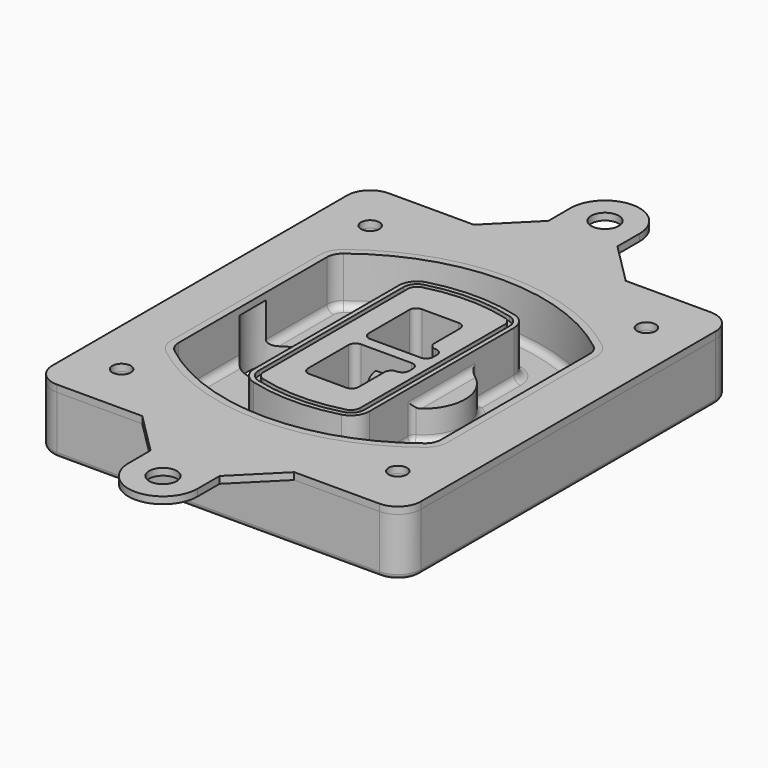
from build123d import *

# Parameters (mm, degrees)
F0_R      = 4
F1_DEPTH  = 25
F2_DEPTH  = 3
F3_DEPTH  = 18
F5_DEPTH  = 21
F6_DEPTH  = 2
F8_DEPTH  = 20
F9_DEPTH  = 16
F10_DEPTH = 25
F7_R      = 6
F7_R_2    = 4
F11_DEPTH = 6
F13_DEPTH = 9
F14_R     = 3
F15_R     = 2
F16_R     = 4
F16_R_2   = 6
F17_DEPTH = 3


# Not quite as in the source:
# - ends of sketch curves that miss each other by under 0.0002 mm in the source are joined


with BuildPart() as f1:
    # F0 (on Top) → F1 (new body)
    with BuildSketch(Plane.XY):
        with BuildLine():
            ThreePointArc((-80, -80), (-77.0710678119, -87.0710678119), (-70, -90))
            Line((-70, -90), (70, -90))
            ThreePointArc((70, -90), (77.0710678119, -87.0710678119), (80, -80))
            Line((80, -80), (80, 80))
            ThreePointArc((80, 80), (77.0710678119, 87.0710678119), (70, 90))
            Line((70, 90), (-70, 90))
            ThreePointArc((-70, 90), (-77.0710678119, 87.0710678119), (-80, 80))
            Line((-80, 80), (-80, -80))
        make_face()
        with Locations((-60, -67.5)):
            Circle(F0_R, mode=Mode.SUBTRACT)
        with Locations((60, -67.5)):
            Circle(F0_R, mode=Mode.SUBTRACT)
        with Locations((-60, 67.5)):
            Circle(F0_R, mode=Mode.SUBTRACT)
        with BuildLine():
            ThreePointArc((-64, 40.2934422872), (-62.5820384798, 46.4328484224), (-58.6153846154, 51.3286200352))
            ThreePointArc((-58.6153846154, 51.3286200352), (0, 71.5), (58.6153846154, 51.3286200352))
            ThreePointArc((58.6153846154, 51.3286200352), (62.5820384798, 46.4328484224), (64, 40.2934422872))
            Line((64, 40.2934422872), (64, -40.2934422872))
            ThreePointArc((64, -40.2934422872), (62.5820384798, -46.4328484224), (58.6153846154, -51.3286200352))
            ThreePointArc((58.6153846154, -51.3286200352), (0, -71.5), (-58.6153846154, -51.3286200352))
            ThreePointArc((-58.6153846154, -51.3286200352), (-62.5820384798, -46.4328484224), (-64, -40.2934422872))
            Line((-64, -40.2934422872), (-64, 40.2934422872))
        make_face(mode=Mode.SUBTRACT)
        with Locations((60, 67.5)):
            Circle(F0_R, mode=Mode.SUBTRACT)
        with BuildLine():
            ThreePointArc((58.6153846154, 51.3286200352), (0, 71.5), (-58.6153846154, 51.3286200352))
            ThreePointArc((-58.6153846154, 51.3286200352), (-62.5820384798, 46.4328484224), (-64, 40.2934422872))
            Line((-64, 40.2934422872), (-64, -40.2934422872))
            ThreePointArc((-64, -40.2934422872), (-62.5820384798, -46.4328484224), (-58.6153846154, -51.3286200352))
            ThreePointArc((-58.6153846154, -51.3286200352), (0, -71.5), (58.6153846154, -51.3286200352))
            ThreePointArc((58.6153846154, -51.3286200352), (62.5820384798, -46.4328484224), (64, -40.2934422872))
            Line((64, -40.2934422872), (64, 40.2934422872))
            ThreePointArc((64, 40.2934422872), (62.5820384798, 46.4328484224), (58.6153846154, 51.3286200352))
        make_face()
        with BuildLine():
            Line((-60, -40.2934422872), (-60, 40.2934422872))
            ThreePointArc((-60, 40.2934422872), (-58.9871703427, 44.6787323838), (-56.1538461538, 48.1757121072))
            ThreePointArc((-56.1538461538, 48.1757121072), (0, 67.5), (56.1538461538, 48.1757121072))
            ThreePointArc((56.1538461538, 48.1757121072), (58.9871703427, 44.6787323838), (60, 40.2934422872))
            Line((60, 40.2934422872), (60, -40.2934422872))
            ThreePointArc((60, -40.2934422872), (58.9871703427, -44.6787323838), (56.1538461538, -48.1757121072))
            ThreePointArc((56.1538461538, -48.1757121072), (0, -67.5), (-56.1538461538, -48.1757121072))
            ThreePointArc((-56.1538461538, -48.1757121072), (-58.9871703427, -44.6787323838), (-60, -40.2934422872))
        make_face(mode=Mode.SUBTRACT)
        with BuildLine():
            ThreePointArc((-56.1538461538, 48.1757121072), (-58.9871703427, 44.6787323838), (-60, 40.2934422872))
            Line((-60, 40.2934422872), (-60, -40.2934422872))
            ThreePointArc((-60, -40.2934422872), (-58.9871703427, -44.6787323838), (-56.1538461538, -48.1757121072))
            ThreePointArc((-56.1538461538, -48.1757121072), (0, -67.5), (56.1538461538, -48.1757121072))
            ThreePointArc((56.1538461538, -48.1757121072), (58.9871703427, -44.6787323838), (60, -40.2934422872))
            Line((60, -40.2934422872), (60, 40.2934422872))
            ThreePointArc((60, 40.2934422872), (58.9871703427, 44.6787323838), (56.1538461538, 48.1757121072))
            ThreePointArc((56.1538461538, 48.1757121072), (0, 67.5), (-56.1538461538, 48.1757121072))
        make_face()
        with BuildLine():
            ThreePointArc((54.3076923077, 45.8110311612), (56.2910192399, 43.3631453548), (57, 40.2934422872))
            Line((57, 40.2934422872), (57, -40.2934422872))
            ThreePointArc((57, -40.2934422872), (56.2910192399, -43.3631453548), (54.3076923077, -45.8110311612))
            ThreePointArc((54.3076923077, -45.8110311612), (0, -64.5), (-54.3076923077, -45.8110311612))
            ThreePointArc((-54.3076923077, -45.8110311612), (-56.2910192399, -43.3631453548), (-57, -40.2934422872))
            Line((-57, -40.2934422872), (-57, 40.2934422872))
            ThreePointArc((-57, 40.2934422872), (-56.2910192399, 43.3631453548), (-54.3076923077, 45.8110311612))
            ThreePointArc((-54.3076923077, 45.8110311612), (0, 64.5), (54.3076923077, 45.8110311612))
        make_face(mode=Mode.SUBTRACT)
        with BuildLine():
            Line((57, -40.2934422872), (57, 40.2934422872))
            ThreePointArc((57, 40.2934422872), (56.2910192399, 43.3631453548), (54.3076923077, 45.8110311612))
            ThreePointArc((54.3076923077, 45.8110311612), (0, 64.5), (-54.3076923077, 45.8110311612))
            ThreePointArc((-54.3076923077, 45.8110311612), (-56.2910192399, 43.3631453548), (-57, 40.2934422872))
            Line((-57, 40.2934422872), (-57, -40.2934422872))
            ThreePointArc((-57, -40.2934422872), (-56.2910192399, -43.3631453548), (-54.3076923077, -45.8110311612))
            ThreePointArc((-54.3076923077, -45.8110311612), (0, -64.5), (54.3076923077, -45.8110311612))
            ThreePointArc((54.3076923077, -45.8110311612), (56.2910192399, -43.3631453548), (57, -40.2934422872))
        make_face()
    extrude(amount=-F1_DEPTH)

    # F0 (on Top) → F2 (join)
    with BuildSketch(Plane.XY):
        with BuildLine():
            ThreePointArc((-56.1538461538, 48.1757121072), (-58.9871703427, 44.6787323838), (-60, 40.2934422872))
            Line((-60, 40.2934422872), (-60, -40.2934422872))
            ThreePointArc((-60, -40.2934422872), (-58.9871703427, -44.6787323838), (-56.1538461538, -48.1757121072))
            ThreePointArc((-56.1538461538, -48.1757121072), (0, -67.5), (56.1538461538, -48.1757121072))
            ThreePointArc((56.1538461538, -48.1757121072), (58.9871703427, -44.6787323838), (60, -40.2934422872))
            Line((60, -40.2934422872), (60, 40.2934422872))
            ThreePointArc((60, 40.2934422872), (58.9871703427, 44.6787323838), (56.1538461538, 48.1757121072))
            ThreePointArc((56.1538461538, 48.1757121072), (0, 67.5), (-56.1538461538, 48.1757121072))
        make_face()
        with BuildLine():
            ThreePointArc((54.3076923077, 45.8110311612), (56.2910192399, 43.3631453548), (57, 40.2934422872))
            Line((57, 40.2934422872), (57, -40.2934422872))
            ThreePointArc((57, -40.2934422872), (56.2910192399, -43.3631453548), (54.3076923077, -45.8110311612))
            ThreePointArc((54.3076923077, -45.8110311612), (0, -64.5), (-54.3076923077, -45.8110311612))
            ThreePointArc((-54.3076923077, -45.8110311612), (-56.2910192399, -43.3631453548), (-57, -40.2934422872))
            Line((-57, -40.2934422872), (-57, 40.2934422872))
            ThreePointArc((-57, 40.2934422872), (-56.2910192399, 43.3631453548), (-54.3076923077, 45.8110311612))
            ThreePointArc((-54.3076923077, 45.8110311612), (0, 64.5), (54.3076923077, 45.8110311612))
        make_face(mode=Mode.SUBTRACT)
    extrude(amount=F2_DEPTH)

    # F0 (on Top) → F3 (cut)
    with BuildSketch(Plane.XY):
        with BuildLine():
            Line((57, -40.2934422872), (57, 40.2934422872))
            ThreePointArc((57, 40.2934422872), (56.2910192399, 43.3631453548), (54.3076923077, 45.8110311612))
            ThreePointArc((54.3076923077, 45.8110311612), (0, 64.5), (-54.3076923077, 45.8110311612))
            ThreePointArc((-54.3076923077, 45.8110311612), (-56.2910192399, 43.3631453548), (-57, 40.2934422872))
            Line((-57, 40.2934422872), (-57, -40.2934422872))
            ThreePointArc((-57, -40.2934422872), (-56.2910192399, -43.3631453548), (-54.3076923077, -45.8110311612))
            ThreePointArc((-54.3076923077, -45.8110311612), (0, -64.5), (54.3076923077, -45.8110311612))
            ThreePointArc((54.3076923077, -45.8110311612), (56.2910192399, -43.3631453548), (57, -40.2934422872))
        make_face()
    extrude(amount=-F3_DEPTH, mode=Mode.SUBTRACT)

    # F4 (on face) → F5 (join, through all)
    with BuildSketch(Plane.XY.offset(3)):
        with BuildLine():
            ThreePointArc((-25, -39.2465276821), (-23.3511545998, -44.1109737193), (-19.0842911877, -46.9702398883))
            ThreePointArc((-19.0842911877, -46.9702398883), (0, -49.5), (19.0842911877, -46.9702398883))
            ThreePointArc((19.0842911877, -46.9702398883), (23.3511545998, -44.1109737193), (25, -39.2465276821))
            Line((25, -39.2465276821), (25, 39.2465276821))
            ThreePointArc((25, 39.2465276821), (23.3511545998, 44.1109737193), (19.0842911877, 46.9702398883))
            ThreePointArc((19.0842911877, 46.9702398883), (0, 49.5), (-19.0842911877, 46.9702398883))
            ThreePointArc((-19.0842911877, 46.9702398883), (-23.3511545998, 44.1109737193), (-25, 39.2465276821))
            Line((-25, 39.2465276821), (-25, -39.2465276821))
        make_face()
        with BuildLine():
            ThreePointArc((18.5632183908, 45.0393118368), (21.7633659499, 42.89486221), (23, 39.2465276821))
            Line((23, 39.2465276821), (23, -39.2465276821))
            ThreePointArc((23, -39.2465276821), (21.7633659499, -42.89486221), (18.5632183908, -45.0393118368))
            ThreePointArc((18.5632183908, -45.0393118368), (0, -47.5), (-18.5632183908, -45.0393118368))
            ThreePointArc((-18.5632183908, -45.0393118368), (-21.7633659499, -42.89486221), (-23, -39.2465276821))
            Line((-23, -39.2465276821), (-23, 39.2465276821))
            ThreePointArc((-23, 39.2465276821), (-21.7633659499, 42.89486221), (-18.5632183908, 45.0393118368))
            ThreePointArc((-18.5632183908, 45.0393118368), (0, 47.5), (18.5632183908, 45.0393118368))
        make_face(mode=Mode.SUBTRACT)
        with BuildLine():
            Line((23, -39.2465276821), (23, 39.2465276821))
            ThreePointArc((23, 39.2465276821), (21.7633659499, 42.89486221), (18.5632183908, 45.0393118368))
            ThreePointArc((18.5632183908, 45.0393118368), (0, 47.5), (-18.5632183908, 45.0393118368))
            ThreePointArc((-18.5632183908, 45.0393118368), (-21.7633659499, 42.89486221), (-23, 39.2465276821))
            Line((-23, 39.2465276821), (-23, -39.2465276821))
            ThreePointArc((-23, -39.2465276821), (-21.7633659499, -42.89486221), (-18.5632183908, -45.0393118368))
            ThreePointArc((-18.5632183908, -45.0393118368), (0, -47.5), (18.5632183908, -45.0393118368))
            ThreePointArc((18.5632183908, -45.0393118368), (21.7633659499, -42.89486221), (23, -39.2465276821))
        make_face()
        with BuildLine():
            ThreePointArc((18.0421455939, 43.1083837852), (20.1755772999, 41.6787507007), (21, 39.2465276821))
            Line((21, 39.2465276821), (21, -39.2465276821))
            ThreePointArc((21, -39.2465276821), (20.1755772999, -41.6787507007), (18.0421455939, -43.1083837852))
            ThreePointArc((18.0421455939, -43.1083837852), (0, -45.5), (-18.0421455939, -43.1083837852))
            ThreePointArc((-18.0421455939, -43.1083837852), (-20.1755772999, -41.6787507007), (-21, -39.2465276821))
            Line((-21, -39.2465276821), (-21, 39.2465276821))
            ThreePointArc((-21, 39.2465276821), (-20.1755772999, 41.6787507007), (-18.0421455939, 43.1083837852))
            ThreePointArc((-18.0421455939, 43.1083837852), (0, 45.5), (18.0421455939, 43.1083837852))
        make_face(mode=Mode.SUBTRACT)
        with BuildLine():
            Line((21, -39.2465276821), (21, 39.2465276821))
            ThreePointArc((21, 39.2465276821), (20.1755772999, 41.6787507007), (18.0421455939, 43.1083837852))
            ThreePointArc((18.0421455939, 43.1083837852), (0, 45.5), (-18.0421455939, 43.1083837852))
            ThreePointArc((-18.0421455939, 43.1083837852), (-20.1755772999, 41.6787507007), (-21, 39.2465276821))
            Line((-21, 39.2465276821), (-21, -39.2465276821))
            ThreePointArc((-21, -39.2465276821), (-20.1755772999, -41.6787507007), (-18.0421455939, -43.1083837852))
            ThreePointArc((-18.0421455939, -43.1083837852), (0, -45.5), (18.0421455939, -43.1083837852))
            ThreePointArc((18.0421455939, -43.1083837852), (20.1755772999, -41.6787507007), (21, -39.2465276821))
        make_face()
        with BuildLine():
            Line((-8, -2.5), (14, -2.5))
            ThreePointArc((14, -2.5), (16.1213203436, -3.3786796564), (17, -5.5))
            Line((17, -5.5), (17, -7.5))
            ThreePointArc((17, -7.5), (16.1213203436, -9.6213203436), (14, -10.5))
            ThreePointArc((14, -10.5), (11.8786796564, -11.3786796564), (11, -13.5))
            Line((11, -13.5), (11, -27.5))
            ThreePointArc((11, -27.5), (10.1213203436, -29.6213203436), (8, -30.5))
            Line((8, -30.5), (-8, -30.5))
            ThreePointArc((-8, -30.5), (-10.1213203436, -29.6213203436), (-11, -27.5))
            Line((-11, -27.5), (-11, -5.5))
            ThreePointArc((-11, -5.5), (-10.1213203436, -3.3786796564), (-8, -2.5))
        make_face(mode=Mode.SUBTRACT)
        with BuildLine():
            ThreePointArc((-8, 2.5), (-10.1213203436, 3.3786796564), (-11, 5.5))
            Line((-11, 5.5), (-11, 27.5))
            ThreePointArc((-11, 27.5), (-10.1213203436, 29.6213203436), (-8, 30.5))
            Line((-8, 30.5), (8, 30.5))
            ThreePointArc((8, 30.5), (10.1213203436, 29.6213203436), (11, 27.5))
            Line((11, 27.5), (11, 13.5))
            ThreePointArc((11, 13.5), (11.8786796564, 11.3786796564), (14, 10.5))
            ThreePointArc((14, 10.5), (16.1213203436, 9.6213203436), (17, 7.5))
            Line((17, 7.5), (17, 5.5))
            ThreePointArc((17, 5.5), (16.1213203436, 3.3786796564), (14, 2.5))
            Line((14, 2.5), (-8, 2.5))
        make_face(mode=Mode.SUBTRACT)
    extrude(amount=-F5_DEPTH)

    # F4 (on face) → F6 (cut)
    with BuildSketch(Plane.XY.offset(3)):
        with BuildLine():
            Line((23, -39.2465276821), (23, 39.2465276821))
            ThreePointArc((23, 39.2465276821), (21.7633659499, 42.89486221), (18.5632183908, 45.0393118368))
            ThreePointArc((18.5632183908, 45.0393118368), (0, 47.5), (-18.5632183908, 45.0393118368))
            ThreePointArc((-18.5632183908, 45.0393118368), (-21.7633659499, 42.89486221), (-23, 39.2465276821))
            Line((-23, 39.2465276821), (-23, -39.2465276821))
            ThreePointArc((-23, -39.2465276821), (-21.7633659499, -42.89486221), (-18.5632183908, -45.0393118368))
            ThreePointArc((-18.5632183908, -45.0393118368), (0, -47.5), (18.5632183908, -45.0393118368))
            ThreePointArc((18.5632183908, -45.0393118368), (21.7633659499, -42.89486221), (23, -39.2465276821))
        make_face()
        with BuildLine():
            ThreePointArc((18.0421455939, 43.1083837852), (20.1755772999, 41.6787507007), (21, 39.2465276821))
            Line((21, 39.2465276821), (21, -39.2465276821))
            ThreePointArc((21, -39.2465276821), (20.1755772999, -41.6787507007), (18.0421455939, -43.1083837852))
            ThreePointArc((18.0421455939, -43.1083837852), (0, -45.5), (-18.0421455939, -43.1083837852))
            ThreePointArc((-18.0421455939, -43.1083837852), (-20.1755772999, -41.6787507007), (-21, -39.2465276821))
            Line((-21, -39.2465276821), (-21, 39.2465276821))
            ThreePointArc((-21, 39.2465276821), (-20.1755772999, 41.6787507007), (-18.0421455939, 43.1083837852))
            ThreePointArc((-18.0421455939, 43.1083837852), (0, 45.5), (18.0421455939, 43.1083837852))
        make_face(mode=Mode.SUBTRACT)
    extrude(amount=-F6_DEPTH, mode=Mode.SUBTRACT)

    # F7 (on face) → F8 (join)
    with BuildSketch(Plane(origin=(0, 0, -25), x_dir=(1, 0, 0), z_dir=(0, 0, -1))):
        with BuildLine():
            ThreePointArc((3.28842436, 0), (16.7567035675, 13.4682792075), (30.224982775, 0))
            Line((30.224982775, 0), (35.224982775, 0))
            ThreePointArc((35.224982775, 0), (16.7567035675, 18.4682792075), (-1.71157564, 0))
            Line((-1.71157564, 0), (3.28842436, 0))
        make_face()
        with BuildLine():
            Line((3.28842436, 0), (30.224982775, 0))
            ThreePointArc((30.224982775, 0), (16.7567035675, 13.4682792075), (3.28842436, 0))
        make_face()
        with BuildLine():
            ThreePointArc((3.28842436, 0), (16.7567035675, -13.4682792075), (30.224982775, 0))
            Line((30.224982775, 0), (3.28842436, 0))
        make_face()
        with BuildLine():
            Line((35.224982775, 0), (30.224982775, 0))
            ThreePointArc((30.224982775, 0), (16.7567035675, -13.4682792075), (3.28842436, 0))
            Line((3.28842436, 0), (-1.71157564, 0))
            ThreePointArc((-1.71157564, 0), (16.7567035675, -18.4682792075), (35.224982775, 0))
        make_face()
    extrude(amount=-F8_DEPTH)

    # F7 (on face) → F9 (cut)
    with BuildSketch(Plane(origin=(0, 0, -25), x_dir=(1, 0, 0), z_dir=(0, 0, -1))):
        with BuildLine():
            Line((3.28842436, 0), (30.224982775, 0))
            ThreePointArc((30.224982775, 0), (16.7567035675, 13.4682792075), (3.28842436, 0))
        make_face()
        with BuildLine():
            ThreePointArc((3.28842436, 0), (16.7567035675, -13.4682792075), (30.224982775, 0))
            Line((30.224982775, 0), (3.28842436, 0))
        make_face()
    extrude(amount=-F9_DEPTH, mode=Mode.SUBTRACT)

    # F7 (on face) → F10 (cut)
    with BuildSketch(Plane(origin=(0, 0, -25), x_dir=(1, 0, 0), z_dir=(0, 0, -1))):
        with BuildLine():
            Line((-59.0318229325, 0), (-32.0952645175, 0))
            ThreePointArc((-32.0952645175, 0), (-45.563543725, 13.4682792075), (-59.0318229325, 0))
        make_face()
        with BuildLine():
            ThreePointArc((-59.0318229325, 0), (-45.563543725, -13.4682792075), (-32.0952645175, 0))
            Line((-32.0952645175, 0), (-59.0318229325, 0))
        make_face()
    extrude(amount=-F10_DEPTH, mode=Mode.SUBTRACT)

    # F7 (on face) → F11 (cut)
    with BuildSketch(Plane(origin=(0, 0, -25), x_dir=(1, 0, 0), z_dir=(0, 0, -1))):
        with Locations((60, -67.5)):
            Circle(F7_R)
        with Locations((60, -67.5)):
            Circle(F7_R_2, mode=Mode.SUBTRACT)
        with Locations((-60, -67.5)):
            Circle(F7_R)
        with Locations((-60, -67.5)):
            Circle(F7_R_2, mode=Mode.SUBTRACT)
        with Locations((-60, 67.5)):
            Circle(F7_R)
        with Locations((-60, 67.5)):
            Circle(F7_R_2, mode=Mode.SUBTRACT)
        with Locations((60, 67.5)):
            Circle(F7_R)
        with Locations((60, 67.5)):
            Circle(F7_R_2, mode=Mode.SUBTRACT)
    extrude(amount=-F11_DEPTH, mode=Mode.SUBTRACT)

    # F12 (on face) → F13 (cut, through all)
    with BuildSketch(Plane(origin=(0, 0, -9), x_dir=(1, 0, 0), z_dir=(0, 0, -1))):
        with BuildLine():
            Line((11, 13.5), (11, 17.5481537753))
            ThreePointArc((11, 17.5481537753), (2.5696536419, 11.8239143813), (-1.5415842455, 2.5))
            Line((-1.5415842455, 2.5), (3.5224848595, 2.5))
            ThreePointArc((3.5224848595, 2.5), (6.1857188154, 8.3455872281), (11.2536447004, 12.2927168648))
            ThreePointArc((11.2536447004, 12.2927168648), (11.0640958889, 12.8831798879), (11, 13.5))
        make_face()
        with BuildLine():
            ThreePointArc((11.2536447004, -12.2927168648), (6.1857188154, -8.3455872281), (3.5224848595, -2.5))
            Line((3.5224848595, -2.5), (-1.5415842455, -2.5))
            ThreePointArc((-1.5415842455, -2.5), (2.5696536419, -11.8239143813), (11, -17.5481537753))
            Line((11, -17.5481537753), (11, -13.5))
            ThreePointArc((11, -13.5), (11.0640958889, -12.8831798879), (11.2536447004, -12.2927168648))
        make_face()
        with BuildLine():
            ThreePointArc((11.2536447004, 12.2927168648), (6.1857188154, 8.3455872281), (3.5224848595, 2.5))
            Line((3.5224848595, 2.5), (14, 2.5))
            ThreePointArc((14, 2.5), (16.1213203436, 3.3786796564), (17, 5.5))
            Line((17, 5.5), (17, 7.5))
            ThreePointArc((17, 7.5), (16.1213203436, 9.6213203436), (14, 10.5))
            ThreePointArc((14, 10.5), (12.3601599782, 10.9878446101), (11.2536447004, 12.2927168648))
        make_face()
        with BuildLine():
            Line((14, -2.5), (3.5224848595, -2.5))
            ThreePointArc((3.5224848595, -2.5), (6.1857188154, -8.3455872281), (11.2536447004, -12.2927168648))
            ThreePointArc((11.2536447004, -12.2927168648), (12.3601599782, -10.9878446101), (14, -10.5))
            ThreePointArc((14, -10.5), (16.1213203436, -9.6213203436), (17, -7.5))
            Line((17, -7.5), (17, -5.5))
            ThreePointArc((17, -5.5), (16.1213203436, -3.3786796564), (14, -2.5))
        make_face()
    extrude(amount=F13_DEPTH, mode=Mode.SUBTRACT)

    # F14
    f14_edges = [f1.edges().sort_by_distance(p)[0] for p in [
        (-57, -23.703476, -18),
        (-57, 23.703476, -18),
        (25, 0, -5),
        (25, 16.526506, -11.5),
        (25, -16.526506, -11.5),
        (25, -27.886517, -18),
        (35.224983, 0, -18),
    ]]
    fillet(f14_edges, radius=F14_R)

    # F15
    f15_edges = [f1.edges().sort_by_distance(p)[0] for p in [
        (0, -90, -25),
    ]]
    fillet(f15_edges, radius=F15_R)


with BuildPart() as f17:
    # F16 (on face) → F17 (new body, through all)
    with BuildSketch(Plane.XY):
        with BuildLine():
            Line((-33, 90), (-70, 90))
            ThreePointArc((-70, 90), (-77.0710678119, 87.0710678119), (-80, 80))
            Line((-80, 80), (-80, -80))
            ThreePointArc((-80, -80), (-77.0710678119, -87.0710678119), (-70, -90))
            Line((-70, -90), (-33, -90))
            Line((-33, -90), (33, -90))
            Line((33, -90), (70, -90))
            ThreePointArc((70, -90), (77.0710678119, -87.0710678119), (80, -80))
            Line((80, -80), (80, 80))
            ThreePointArc((80, 80), (77.0710678119, 87.0710678119), (70, 90))
            Line((70, 90), (33, 90))
            Line((33, 90), (-33, 90))
        make_face()
        with Locations((-60, -67.5)):
            Circle(F16_R, mode=Mode.SUBTRACT)
        with Locations((60, -67.5)):
            Circle(F16_R, mode=Mode.SUBTRACT)
        with Locations((-60, 67.5)):
            Circle(F16_R, mode=Mode.SUBTRACT)
        with BuildLine():
            ThreePointArc((-56.1538461538, 48.1757121072), (0, 67.5), (56.1538461538, 48.1757121072))
            ThreePointArc((56.1538461538, 48.1757121072), (58.9871703427, 44.6787323838), (60, 40.2934422872))
            Line((60, 40.2934422872), (60, -40.2934422872))
            ThreePointArc((60, -40.2934422872), (58.9871703427, -44.6787323838), (56.1538461538, -48.1757121072))
            ThreePointArc((56.1538461538, -48.1757121072), (0, -67.5), (-56.1538461538, -48.1757121072))
            ThreePointArc((-56.1538461538, -48.1757121072), (-58.9871703427, -44.6787323838), (-60, -40.2934422872))
            Line((-60, -40.2934422872), (-60, 40.2934422872))
            ThreePointArc((-60, 40.2934422872), (-58.9871703427, 44.6787323838), (-56.1538461538, 48.1757121072))
        make_face(mode=Mode.SUBTRACT)
        with Locations((60, 67.5)):
            Circle(F16_R, mode=Mode.SUBTRACT)
        with BuildLine():
            Line((-15, 107.999997735), (-33, 89.999997735))
            Line((-33, 89.999997735), (33, 90))
            Line((33, 90), (15, 107.999997735))
            Line((15, 107.999997735), (15, 119.999997735))
            ThreePointArc((15, 119.999997735), (0, 134.999997735), (-15, 119.999997735))
            Line((-15, 119.999997735), (-15, 107.999997735))
        make_face()
        with Locations((0, 119.999997735)):
            Circle(F16_R_2, mode=Mode.SUBTRACT)
        with BuildLine():
            Line((33, -90), (-33, -90))
            Line((-33, -90), (-15, -107.999997735))
            Line((-15, -107.999997735), (-15, -119.999997735))
            ThreePointArc((-15, -119.999997735), (0, -134.999997735), (15, -119.999997735))
            Line((15, -119.999997735), (15, -107.999997735))
            Line((15, -107.999997735), (33, -90))
        make_face()
        with Locations((0, -119.999997735)):
            Circle(F16_R_2, mode=Mode.SUBTRACT)
    extrude(amount=F17_DEPTH)


solid = Compound([f1.part, f17.part])
